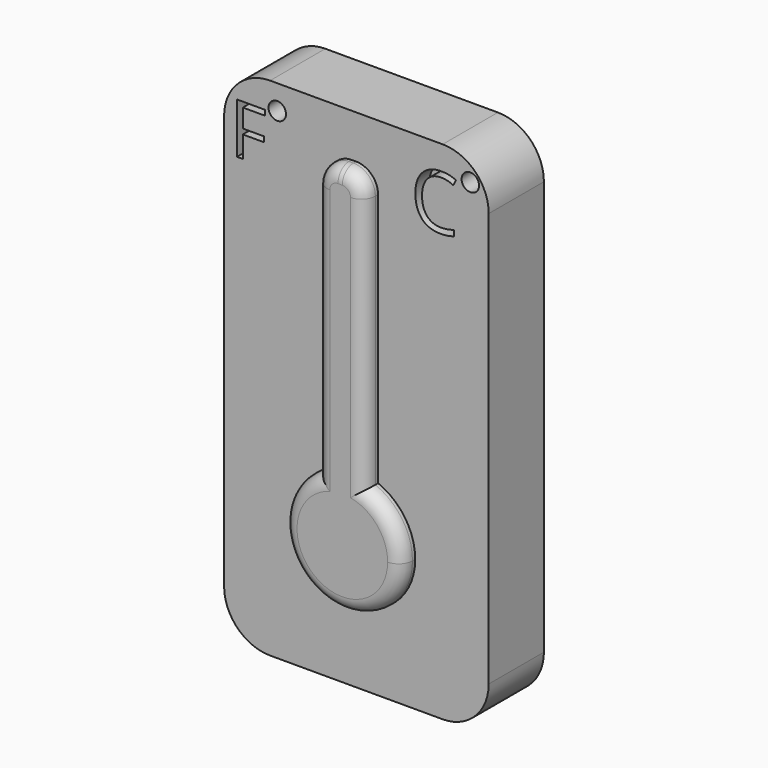
from build123d import *

# Parameters (mm, degrees)
F1_DEPTH       = 25.4
F2_R           = 3.2131
F2_TEXT_SIZE   = 26.0304922276
F2_TEXT_SIZE_2 = 27.7123537124
F3_DEPTH       = 6.35
F4_DEPTH       = 12.7
F5_R           = 5.08


# Not quite as in the source:
# - Text() gives the source's letters only with a copy of the font that has no kerning and outlines rounded to 1/6400 em; it was checked with that copy


with BuildPart() as f1:
    # F0 (on Front) → F1 (new body)
    with BuildSketch(Plane.XZ):
        with BuildLine():
            Line((31.8496580859, 92.2875252639), (-31.6503419141, 92.2875252639))
            ThreePointArc((-31.6503419141, 92.2875252639), (-43.6240167422, 87.3278667586), (-48.5836752474, 75.3541919305))
            Line((-48.5836752474, 75.3541919305), (-48.5836752474, -77.0458080695))
            ThreePointArc((-48.5836752474, -77.0458080695), (-43.6240167422, -89.0194828976), (-31.6503419141, -93.9791414028))
            Line((-31.6503419141, -93.9791414028), (31.8496580859, -93.9791414028))
            ThreePointArc((31.8496580859, -93.9791414028), (43.823332914, -89.0194828976), (48.7829914192, -77.0458080695))
            Line((48.7829914192, -77.0458080695), (48.7829914192, 75.3541919305))
            ThreePointArc((48.7829914192, 75.3541919305), (43.823332914, 87.3278667586), (31.8496580859, 92.2875252639))
        make_face()
    extrude(amount=F1_DEPTH)

    # F2 (on face) → F3 (cut)
    with BuildSketch(Plane.XZ.offset(25.4)):
        with Locations((42.0337234153, 83.2936468059)):
            Circle(F2_R)
        with Locations((-29.0235932916, 83.3177119493)):
            Circle(F2_R)
        with BuildLine():
            Line((0.0045861115, 76.3600636364), (-1.6005784937, 76.3600636364))
            ThreePointArc((-1.6005784937, 76.3600636364), (-7.3155784937, 73.9928331275), (-9.6828090027, 68.2778331275))
            Line((-9.6828090027, 68.2778331275), (-9.6828090027, -25.937604359))
            ThreePointArc((-9.6828090027, -25.937604359), (-0.8744277251, -23.6806989203), (8.0868166204, -25.2225493253))
            Line((8.0868166204, -25.2225493253), (8.0868166204, 68.2778331275))
            ThreePointArc((8.0868166204, 68.2778331275), (5.7195861115, 73.9928331275), (0.0045861115, 76.3600636364))
        make_face()
        with BuildLine():
            ThreePointArc((8.0868166204, -25.2225493253), (-0.8744277251, -23.6806989203), (-9.6828090027, -25.937604359))
            Line((-9.6828090027, -25.937604359), (-9.6828090027, -53.811184845))
            Line((-9.6828090027, -53.811184845), (8.0868166204, -53.811184845))
            Line((8.0868166204, -53.811184845), (8.0868166204, -25.2225493253))
        make_face()
        with BuildLine():
            Line((-9.6828090027, -53.811184845), (-9.6828090027, -25.937604359))
            ThreePointArc((-9.6828090027, -25.937604359), (-11.4539266629, -63.8979153633), (21.7477367334, -45.410849154))
            ThreePointArc((21.7477367334, -45.410849154), (18.0115797739, -33.222861335), (8.0868166204, -25.2225493253))
            Line((8.0868166204, -25.2225493253), (8.0868166204, -53.811184845))
            Line((8.0868166204, -53.811184845), (-9.6828090027, -53.811184845))
        make_face()
        with Locations((-46.4059533, 63.6319552484)):
            Text('F', F2_TEXT_SIZE, font='Open Sans', text_align=(TextAlign.LEFT, TextAlign.BOTTOM))
        with Locations((20.1091005581, 63.340752133)):
            Text('C', F2_TEXT_SIZE_2, font='Open Sans', text_align=(TextAlign.LEFT, TextAlign.BOTTOM))
    extrude(amount=-F3_DEPTH, mode=Mode.SUBTRACT)

    # F4 (add): a face of the model
    f4_faces = [f1.faces().sort_by_distance(p)[0] for p in [
        (-0.4383515736, -19.05, -7.0869816291),
    ]]
    extrude(f4_faces, amount=F4_DEPTH)

    # F5
    f5_edges = [f1.edges().sort_by_distance(p)[0] for p in [
        (-9.682809, -31.75, 21.170114),
        (5.719586, -31.75, 73.992833),
        (-0.797996, -31.75, 76.360064),
        (-7.315578, -31.75, 73.992833),
        (0.874428, -31.75, -67.140999),
        (8.086817, -31.75, 21.527642),
    ]]
    fillet(f5_edges, radius=F5_R)


solid = f1.part
